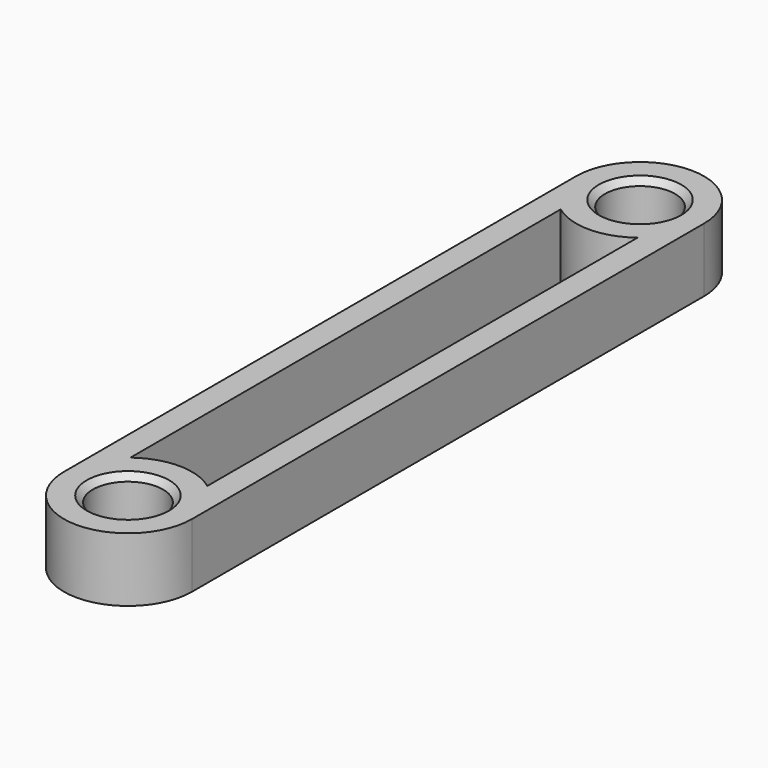
from build123d import *

# Parameters (mm, degrees)
F2_R     = 3.4798
F3_DEPTH = 6.35
F4_SIZE2 = 0.6096
F4_SIZE  = 0.6096


# Not quite as in the source:
# - a variable given as a bare number and used for a length is read in inches; the dataset says mm whatever the document's units were


with BuildPart() as f3:
    # F2 (on Top) → F3 (new body)
    with BuildSketch(Plane.XY):
        with BuildLine():
            ThreePointArc((-3.81, -5.08), (-5.6796126628, -2.8398063314), (-6.35, 0))
            Line((-6.35, 0), (-6.35, -63.5))
            ThreePointArc((-6.35, -63.5), (-5.6796126628, -60.6601936686), (-3.81, -58.42))
            Line((-3.81, -58.42), (-3.81, -5.08))
        make_face()
        with BuildLine():
            ThreePointArc((3.81, -5.08), (5.6796126628, -2.8398063314), (6.35, 0))
            ThreePointArc((6.35, 0), (0, 6.35), (-6.35, 0))
            ThreePointArc((-6.35, 0), (-5.6796126628, -2.8398063314), (-3.81, -5.08))
            ThreePointArc((-3.81, -5.08), (0, -6.35), (3.81, -5.08))
        make_face()
        Circle(F2_R, mode=Mode.SUBTRACT)
        with BuildLine():
            Line((6.35, -63.5), (6.35, 0))
            ThreePointArc((6.35, 0), (5.6796126628, -2.8398063314), (3.81, -5.08))
            Line((3.81, -5.08), (3.81, -58.42))
            ThreePointArc((3.81, -58.42), (5.6796126628, -60.6601936686), (6.35, -63.5))
        make_face()
        with BuildLine():
            ThreePointArc((-6.35, -63.5), (0, -69.85), (6.35, -63.5))
            ThreePointArc((6.35, -63.5), (5.6796126628, -60.6601936686), (3.81, -58.42))
            ThreePointArc((3.81, -58.42), (0, -57.15), (-3.81, -58.42))
            ThreePointArc((-3.81, -58.42), (-5.6796126628, -60.6601936686), (-6.35, -63.5))
        make_face()
        with Locations((0, -63.5)):
            Circle(F2_R, mode=Mode.SUBTRACT)
    extrude(amount=F3_DEPTH)

    # F4
    f4_edges = [f3.edges().sort_by_distance(p)[0] for p in [
        (-3.4798, 0, 6.35),
        (-3.4798, -63.5, 6.35),
        (-3.4798, 0, 0),
        (-3.4798, -63.5, 0),
    ]]
    chamfer(f4_edges, length=F4_SIZE, length2=F4_SIZE2)


solid = f3.part
